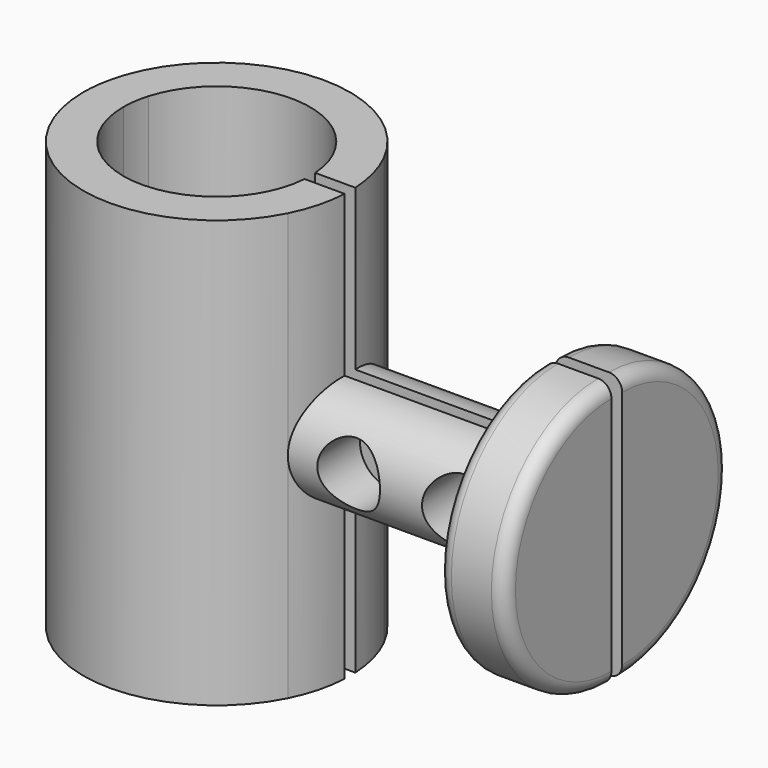
from build123d import *

# Parameters (mm, degrees)
F1_DEPTH      = 16
F3_ANGLE_BACK = 90
F3_ANGLE      = 180
F4_ANGLE_BACK = 90
F4_ANGLE      = 180
F5_R          = 2.34997
F5_R_2        = 2.5
F6_DEPTH      = 20


with BuildPart() as f1:
    # F0 (on Top) → F1 (new body, symmetric)
    with BuildSketch(Plane.XY):
        with BuildLine():
            ThreePointArc((6.92785, 4.5), (7.715866, 2.510323), (6.98212, 0.5))
            Line((6.98212, 0.5), (9.987492, 0.5))
            ThreePointArc((9.987492, 0.5), (9.668018, 2.555273), (8.930286, 4.5))
            Line((8.930286, 4.5), (6.92785, 4.5))
        make_face()
        with BuildLine():
            ThreePointArc((-7, 0), (-6.926667, 1.010587), (-6.708204, 2))
            Line((-6.708204, 2), (-9.797959, 2))
            ThreePointArc((-9.797959, 2), (-9.949362, 1.00509), (-10, 0))
            Line((-10, 0), (-7, 0))
        make_face()
        with BuildLine():
            Line((9.987492, -0.5), (6.98212, -0.5))
            ThreePointArc((6.98212, -0.5), (7.715866, -2.510323), (6.92785, -4.5))
            Line((6.92785, -4.5), (8.930286, -4.5))
            ThreePointArc((8.930286, -4.5), (9.668018, -2.555273), (9.987492, -0.5))
        make_face()
        with BuildLine():
            ThreePointArc((6.92785, -4.5), (7.715866, -2.510323), (6.98212, -0.5))
            ThreePointArc((6.98212, -0.5), (-0.25016, -6.995529), (-7, 0))
            Line((-7, 0), (-10, 0))
            ThreePointArc((-10, 0), (-2.312698, -9.728897), (8.930286, -4.5))
            Line((8.930286, -4.5), (6.92785, -4.5))
        make_face()
        with BuildLine():
            ThreePointArc((-6.708204, 2), (0.762402, 6.958358), (6.98212, 0.5))
            ThreePointArc((6.98212, 0.5), (7.715866, 2.510323), (6.92785, 4.5))
            Line((6.92785, 4.5), (8.930286, 4.5))
            ThreePointArc((8.930286, 4.5), (-1.323146, 9.912078), (-9.797959, 2))
            Line((-9.797959, 2), (-6.708204, 2))
        make_face()
    extrude(amount=F1_DEPTH, both=True)

    # F0 (on Top) → F2 (revolve)
    with BuildSketch(Plane.XY):
        with BuildLine():
            ThreePointArc((-7, 0), (-6.926667, 1.010587), (-6.708204, 2))
            Line((-6.708204, 2), (-9.797959, 2))
            ThreePointArc((-9.797959, 2), (-9.949362, 1.00509), (-10, 0))
            Line((-10, 0), (-7, 0))
        make_face()
        with BuildLine():
            Line((2.291796, 2), (-6.708204, 2))
            ThreePointArc((-6.708204, 2), (-6.926667, 1.010587), (-7, 0))
            Line((-7, 0), (3.291796, 0))
            Line((3.291796, 0), (3.291796, 1))
            ThreePointArc((3.291796, 1), (2.998903, 1.707107), (2.291796, 2))
        make_face()
    revolve(axis=Axis((-3.354102, 0, 0), (-1, 0, 0)))

    # F0 (on Top) → F3 (revolve)
    with BuildSketch(Plane.XY, mode=Mode.PRIVATE) as f3_sk:
        with BuildLine():
            ThreePointArc((6.92785, 4.5), (7.715866, 2.510323), (6.98212, 0.5))
            Line((6.98212, 0.5), (9.987492, 0.5))
            ThreePointArc((9.987492, 0.5), (9.668018, 2.555273), (8.930286, 4.5))
            Line((8.930286, 4.5), (6.92785, 4.5))
        make_face()
        with BuildLine():
            ThreePointArc((8.930286, 4.5), (9.668018, 2.555273), (9.987492, 0.5))
            Line((9.987492, 0.5), (24.987492, 0.5))
            Line((24.987492, 0.5), (24.987492, 4.5))
            Line((24.987492, 4.5), (8.930286, 4.5))
        make_face()
        with BuildLine():
            Line((24.987492, 4.5), (24.987492, 0.5))
            Line((24.987492, 0.5), (29.987492, 0.5))
            Line((29.987492, 0.5), (29.987492, 9.5))
            ThreePointArc((29.987492, 9.5), (29.694599, 10.207107), (28.987492, 10.5))
            Line((28.987492, 10.5), (25.987492, 10.5))
            ThreePointArc((25.987492, 10.5), (25.280385, 10.207107), (24.987492, 9.5))
            Line((24.987492, 9.5), (24.987492, 4.5))
        make_face()
    revolve(f3_sk.sketch.rotate(Axis((17.487492, 0.5, 0), (1, 0, 0)), -F3_ANGLE_BACK), axis=Axis((17.487492, 0.5, 0), (1, 0, 0)), revolution_arc=F3_ANGLE)

    # F0 (on Top) → F4 (revolve)
    with BuildSketch(Plane.XY, mode=Mode.PRIVATE) as f4_sk:
        with BuildLine():
            Line((24.987492, -0.5), (9.987492, -0.5))
            ThreePointArc((9.987492, -0.5), (9.668018, -2.555273), (8.930286, -4.5))
            Line((8.930286, -4.5), (24.987492, -4.5))
            Line((24.987492, -4.5), (24.987492, -0.5))
        make_face()
        with BuildLine():
            Line((29.987492, -0.5), (24.987492, -0.5))
            Line((24.987492, -0.5), (24.987492, -4.5))
            Line((24.987492, -4.5), (24.987492, -9.5))
            ThreePointArc((24.987492, -9.5), (25.280385, -10.207107), (25.987492, -10.5))
            Line((25.987492, -10.5), (28.987492, -10.5))
            ThreePointArc((28.987492, -10.5), (29.694599, -10.207107), (29.987492, -9.5))
            Line((29.987492, -9.5), (29.987492, -0.5))
        make_face()
        with BuildLine():
            Line((9.987492, -0.5), (6.98212, -0.5))
            ThreePointArc((6.98212, -0.5), (7.715866, -2.510323), (6.92785, -4.5))
            Line((6.92785, -4.5), (8.930286, -4.5))
            ThreePointArc((8.930286, -4.5), (9.668018, -2.555273), (9.987492, -0.5))
        make_face()
    revolve(f4_sk.sketch.rotate(Axis((17.487492, -0.5, 0), (1, 0, 0)), -F4_ANGLE_BACK), axis=Axis((17.487492, -0.5, 0), (1, 0, 0)), revolution_arc=F4_ANGLE)

    # F5 (on Front) → F6 (cut, symmetric)
    with BuildSketch(Plane.XZ):
        with Locations((13.487492, 0)):
            Circle(F5_R)
        with Locations((21.487492, 0)):
            Circle(F5_R_2)
    extrude(amount=F6_DEPTH, both=True, mode=Mode.SUBTRACT)


solid = f1.part
